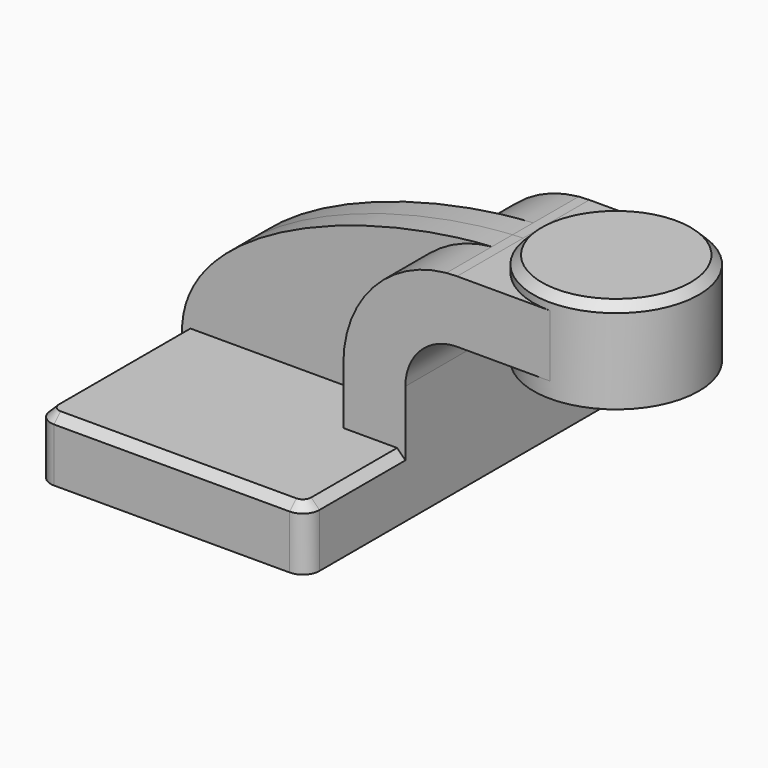
from build123d import *

# Parameters (mm, degrees)
F1_DEPTH     = 63.5
F0_W         = 25.4
F0_H         = 19.05
F2_DEPTH     = 25.4
F3_DEPTH     = 7.9375
F5_R         = 5.08
F6_T1_DEPTH  = 72.39
F6_T3_DEPTH  = 33.02
F6_T5_DEPTH  = 50.4825
F6_T10_ANGLE = 90
F6_T12_ANGLE = 90


# Not quite as in the source:
# - a fillet or chamfer that OpenCascade refuses, or shapes differently, is made with other operations: its cross-section is extruded or revolved along the edge and cut away or added


with BuildPart() as f1:
    # F0 (on Front) → F1 (new body, symmetric)
    with BuildSketch(Plane.XZ):
        Polygon((22.225, 9.525), (-41.275, 9.525), (-41.275, -9.525), (41.275, -9.525), (41.275, 9.525), align=None)
    extrude(amount=F1_DEPTH, both=True)

    # F0 (on Front) → F2 (join, symmetric)
    with BuildSketch(Plane.XZ):
        with BuildLine():
            Line((22.225, 27.0002), (22.225, 9.525))
            Line((22.225, 9.525), (41.275, 9.525))
            Line((41.275, 9.525), (41.275, 27.0002))
            ThreePointArc((41.275, 27.0002), (45.9246798487, 38.2255201513), (57.15, 42.8752))
            Line((57.15, 42.8752), (60.325, 42.8752))
            Line((60.325, 42.8752), (60.325, 61.9252))
            Line((60.325, 61.9252), (57.15, 61.9252))
            add(Edge.make_bspline(
                [(53.8854342407, 61.7722898912), (54.9842067368, 61.8365871986), (56.0728453275, 61.8876096574), (57.15, 61.9252)],
                knots=[108.5245810491, 108.5245810491, 108.5245810491, 108.5245810491, 111.5045361635, 111.5045361635, 111.5045361635, 111.5045361635], degree=3))
            ThreePointArc((53.8854342407, 61.7722898912), (31.3258777096, 50.5133948686), (22.225, 27.0002))
        make_face()
        with Locations((73.025, 52.4002)):
            Rectangle(F0_W, F0_H)
    extrude(amount=F2_DEPTH, both=True)

    # F0 (on Front) → F3 (join, symmetric)
    with BuildSketch(Plane.XZ):
        with BuildLine():
            add(Edge.make_bspline(
                [(-41.275, 9.525), (-39.5856284224, 39.4828766469), (13.870125209, 59.4306981306), (53.8854342407, 61.7722898912)],
                knots=[0, 0, 0, 0, 108.5245810491, 108.5245810491, 108.5245810491, 108.5245810491], degree=3))
            Line((-41.275, 9.525), (22.225, 9.525))
            Line((22.225, 9.525), (22.225, 27.0002))
            ThreePointArc((22.225, 27.0002), (31.3258777096, 50.5133948686), (53.8854342407, 61.7722898912))
        make_face()
    extrude(amount=F3_DEPTH, both=True)

    # F0 (on Front) → F4 (revolve)
    with BuildSketch(Plane.XZ):
        Polygon((85.725, 66.675), (85.725, 61.9252), (85.725, 42.8752), (85.725, 38.1), (111.125, 38.1), (111.125, 66.675), align=None)
    revolve(axis=Axis((85.725, 0, 52.3875), (0, 0, 1)))

    # F5
    f5_edges = [f1.edges().sort_by_distance(p)[0] for p in [
        (41.275, -63.5, 0),
        (-41.275, -63.5, 0),
        (41.275, 63.5, 0),
        (-41.275, 63.5, 0),
    ]]
    fillet(f5_edges, radius=F5_R)

    # F6: chamfer of 2.54 on 6 edges, made by hand

    # F6_s2 → F6_t1 (cut)
    with BuildSketch(Plane.YZ.offset(-36.195)):
        Polygon((-60.96, 9.525), (-63.5, 6.985), (-63.5, 9.525), align=None)
    extrude(amount=F6_T1_DEPTH, mode=Mode.SUBTRACT)

    # F6_s4 → F6_t3 (cut)
    with BuildSketch(Plane.XZ.offset(25.4)):
        Polygon((41.275, 6.985), (38.735, 9.525), (41.275, 9.525), align=None)
    extrude(amount=F6_T3_DEPTH, mode=Mode.SUBTRACT)

    # F6_s6 → F6_t5 (cut)
    with BuildSketch(Plane.XZ.offset(7.9375)):
        Polygon((-41.275, 6.985), (-38.735, 9.525), (-41.275, 9.525), align=None)
    extrude(amount=F6_T5_DEPTH, mode=Mode.SUBTRACT)

    # F6_s7 → F6_t8 (revolve, cut)
    with BuildSketch(Plane.XZ):
        Polygon((111.125, 64.135), (108.585, 66.675), (111.125, 66.675), align=None)
    revolve(axis=Axis((85.725, 0, 66.675), (0, 0, 1)), mode=Mode.SUBTRACT)

    # F6_s9 → F6_t10 (revolve, cut)
    with BuildSketch(Plane.XZ.offset(58.42)):
        Polygon((41.275, 6.985), (38.735, 9.525), (41.275, 9.525), align=None)
    revolve(axis=Axis((36.195, -58.42, 9.525), (0, 0, -1)), revolution_arc=F6_T10_ANGLE, mode=Mode.SUBTRACT)

    # F6_s11 → F6_t12 (revolve, cut)
    with BuildSketch(Plane.XZ.offset(58.42)):
        Polygon((-38.735, 9.525), (-41.275, 6.985), (-41.275, 9.525), align=None)
    revolve(axis=Axis((-36.195, -58.42, 9.525), (0, 0, 1)), revolution_arc=F6_T12_ANGLE, mode=Mode.SUBTRACT)


solid = f1.part
